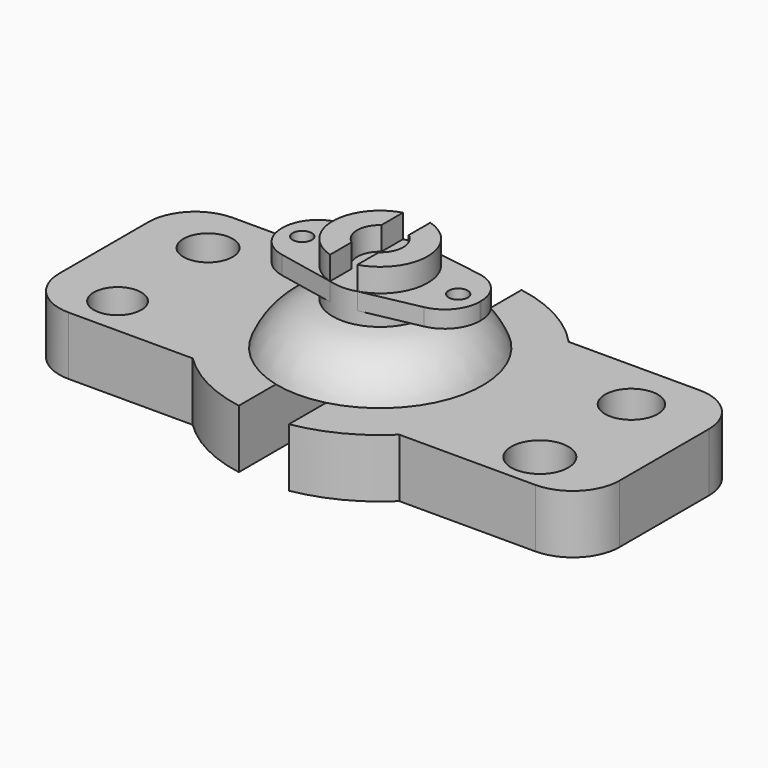
from build123d import *
from build123d import SkipClean  # not in build123d's __all__

# Parameters (mm, degrees)
F0_R      = 10.1568223354
F0_R_2    = 10.5169255504
F0_R_3    = 12.1759626717
F0_R_4    = 11.2592738499
F1_DEPTH  = 25
F2_R      = 20
F3_R      = 20
F4_R      = 20
F5_R      = 20
F6_DEPTH  = 84.25
F7_DEPTH  = 100
F8_DEPTH  = 95.25
F9_DEPTH  = 74.75
F14_DEPTH = 10
F15_DEPTH = 10
F16_DEPTH = 10
F17_DEPTH = 10
F18_DEPTH = 10
F19_R     = 4.0591498716
F20_DEPTH = 7.75
F21_R     = 15
F22_R     = 15
F23_DEPTH = 7.25
F24_R     = 15


with BuildPart() as f1:
    # F0 (on Top) → F1 (new body)
    with BuildSketch(Plane.XY):
        with BuildLine():
            Line((-46.3593495633, 42.660780251), (-117.1441823244, 42.660780251))
            Line((-117.1441823244, 42.660780251), (-117.1441823244, -44.9667572975))
            Line((-117.1441823244, -44.9667572975), (-44.1262076515, -44.9667572975))
            ThreePointArc((-44.1262076515, -44.9667572975), (-62.9805950299, -1.6050274871), (-46.3593495633, 42.660780251))
        make_face()
        with Locations((-89.4723236561, -28.3636450768)):
            Circle(F0_R, mode=Mode.SUBTRACT)
        with Locations((-89.9335220456, 20.5232948065)):
            Circle(F0_R_2, mode=Mode.SUBTRACT)
        with BuildLine():
            ThreePointArc((-10.7280304655, 62.0809215934), (-30.1500864357, 55.3182045215), (-46.3593495633, 42.660780251))
            Line((-46.3593495633, 42.660780251), (-10.7280304655, 42.660780251))
            Line((-10.7280304655, 42.660780251), (-10.7280304655, 62.0809215934))
        make_face()
        with BuildLine():
            Line((-10.7280304655, 42.660780251), (-46.3593495633, 42.660780251))
            ThreePointArc((-46.3593495633, 42.660780251), (-62.9805950299, -1.6050274871), (-44.1262076515, -44.9667572975))
            Line((-44.1262076515, -44.9667572975), (-10.7280304655, -44.9667572975))
            Line((-10.7280304655, -44.9667572975), (-10.7280304655, 42.660780251))
        make_face()
        with BuildLine():
            Line((-10.7280304655, 62.0809215934), (-10.7280304655, 42.660780251))
            Line((-10.7280304655, 42.660780251), (10.6815285981, 42.660780251))
            Line((10.6815285981, 42.660780251), (10.6815285981, 62.0889395172))
            ThreePointArc((10.6815285981, 62.0889395172), (-0.0235940182, 63.0010389349), (-10.7280304655, 62.0809215934))
        make_face()
        with BuildLine():
            Line((-10.7280304655, 68.533860147), (-10.7280304655, 62.0809215934))
            ThreePointArc((-10.7280304655, 62.0809215934), (-0.0235940182, 63.0010389349), (10.6815285981, 62.0889395172))
            Line((10.6815285981, 62.0889395172), (10.6815285981, 68.533860147))
            Line((10.6815285981, 68.533860147), (-10.7280304655, 68.533860147))
        make_face()
        with BuildLine():
            Line((-10.7280304655, -44.9667572975), (-44.1262076515, -44.9667572975))
            ThreePointArc((-44.1262076515, -44.9667572975), (-28.7310026755, -56.0683596052), (-10.7280304655, -62.0809215934))
            Line((-10.7280304655, -62.0809215934), (-10.7280304655, -44.9667572975))
        make_face()
        with BuildLine():
            Line((10.6815285981, 62.0889395172), (10.6815285981, 42.660780251))
            Line((10.6815285981, 42.660780251), (46.3593495633, 42.660780251))
            ThreePointArc((46.3593495633, 42.660780251), (30.1293675419, 55.3294919106), (10.6815285981, 62.0889395172))
        make_face()
        with BuildLine():
            Line((46.3593495633, 42.660780251), (10.6815285981, 42.660780251))
            Line((10.6815285981, 42.660780251), (10.6815285981, -44.9667572975))
            Line((10.6815285981, -44.9667572975), (44.1262076515, -44.9667572975))
            ThreePointArc((44.1262076515, -44.9667572975), (58.0910000982, -24.3837480948), (63.0010433529, 0))
            ThreePointArc((63.0010433529, 0), (58.6933507955, 22.8958956137), (46.3593495633, 42.660780251))
        make_face()
        with BuildLine():
            Line((10.6815285981, -44.9667572975), (-10.7280304655, -44.9667572975))
            Line((-10.7280304655, -44.9667572975), (-10.7280304655, -62.0809215934))
            ThreePointArc((-10.7280304655, -62.0809215934), (-0.0235940182, -63.0010389349), (10.6815285981, -62.0889395172))
            Line((10.6815285981, -62.0889395172), (10.6815285981, -44.9667572975))
        make_face()
        with BuildLine():
            ThreePointArc((10.6815285981, -62.0889395172), (-0.0235940182, -63.0010389349), (-10.7280304655, -62.0809215934))
            Line((-10.7280304655, -62.0809215934), (-10.7280304655, -71.3264122605))
            Line((-10.7280304655, -71.3264122605), (10.6815285981, -71.3264122605))
            Line((10.6815285981, -71.3264122605), (10.6815285981, -62.0889395172))
        make_face()
        with BuildLine():
            Line((122.2173571587, 42.660780251), (46.3593495633, 42.660780251))
            ThreePointArc((46.3593495633, 42.660780251), (58.6933507955, 22.8958956137), (63.0010433529, 0))
            ThreePointArc((63.0010433529, 0), (58.0910000982, -24.3837480948), (44.1262076515, -44.9667572975))
            Line((44.1262076515, -44.9667572975), (122.2173571587, -44.9667572975))
            Line((122.2173571587, -44.9667572975), (122.2173571587, 42.660780251))
        make_face()
        with Locations((90.8559188247, -28.3636450768)):
            Circle(F0_R_3, mode=Mode.SUBTRACT)
        with Locations((90.8559188247, 20.5232948065)):
            Circle(F0_R_4, mode=Mode.SUBTRACT)
        with BuildLine():
            Line((44.1262076515, -44.9667572975), (10.6815285981, -44.9667572975))
            Line((10.6815285981, -44.9667572975), (10.6815285981, -62.0889395172))
            ThreePointArc((10.6815285981, -62.0889395172), (28.7100029466, -56.079115492), (44.1262076515, -44.9667572975))
        make_face()
    extrude(amount=F1_DEPTH)

    # F2
    f2_edges = [f1.edges().sort_by_distance(p)[0] for p in [
        (-117.144182, -44.966757, 12.5),
    ]]
    fillet(f2_edges, radius=F2_R)

    # F3
    f3_edges = [f1.edges().sort_by_distance(p)[0] for p in [
        (-117.144182, 42.66078, 12.5),
    ]]
    fillet(f3_edges, radius=F3_R)

    # F4
    f4_edges = [f1.edges().sort_by_distance(p)[0] for p in [
        (122.217357, 42.66078, 12.5),
    ]]
    fillet(f4_edges, radius=F4_R)

    # F5
    f5_edges = [f1.edges().sort_by_distance(p)[0] for p in [
        (122.217357, -44.966757, 12.5),
    ]]
    fillet(f5_edges, radius=F5_R)

    # F0 (on Top) → F6 (cut)
    with BuildSketch(Plane.XY):
        with BuildLine():
            Line((-10.7280304655, 68.533860147), (-10.7280304655, 62.0809215934))
            ThreePointArc((-10.7280304655, 62.0809215934), (-0.0235940182, 63.0010389349), (10.6815285981, 62.0889395172))
            Line((10.6815285981, 62.0889395172), (10.6815285981, 68.533860147))
            Line((10.6815285981, 68.533860147), (-10.7280304655, 68.533860147))
        make_face()
    with SkipClean():  # cleaning this boolean's faces spoils the solid; the shape is the same uncleaned
        extrude(amount=F6_DEPTH, mode=Mode.SUBTRACT)

    # F0 (on Top) → F7 (cut)
    with BuildSketch(Plane.XY):
        with BuildLine():
            Line((-10.7280304655, 62.0809215934), (-10.7280304655, 42.660780251))
            Line((-10.7280304655, 42.660780251), (10.6815285981, 42.660780251))
            Line((10.6815285981, 42.660780251), (10.6815285981, 62.0889395172))
            ThreePointArc((10.6815285981, 62.0889395172), (-0.0235940182, 63.0010389349), (-10.7280304655, 62.0809215934))
        make_face()
    extrude(amount=F7_DEPTH, mode=Mode.SUBTRACT)

    # F0 (on Top) → F8 (cut)
    with BuildSketch(Plane.XY):
        with BuildLine():
            Line((10.6815285981, -44.9667572975), (-10.7280304655, -44.9667572975))
            Line((-10.7280304655, -44.9667572975), (-10.7280304655, -62.0809215934))
            ThreePointArc((-10.7280304655, -62.0809215934), (-0.0235940182, -63.0010389349), (10.6815285981, -62.0889395172))
            Line((10.6815285981, -62.0889395172), (10.6815285981, -44.9667572975))
        make_face()
    extrude(amount=F8_DEPTH, mode=Mode.SUBTRACT)

    # F0 (on Top) → F9 (cut)
    with BuildSketch(Plane.XY):
        with BuildLine():
            ThreePointArc((10.6815285981, -62.0889395172), (-0.0235940182, -63.0010389349), (-10.7280304655, -62.0809215934))
            Line((-10.7280304655, -62.0809215934), (-10.7280304655, -71.3264122605))
            Line((-10.7280304655, -71.3264122605), (10.6815285981, -71.3264122605))
            Line((10.6815285981, -71.3264122605), (10.6815285981, -62.0889395172))
        make_face()
    extrude(amount=F9_DEPTH, mode=Mode.SUBTRACT)


with BuildPart() as f11:
    # F10 (on Right) → F11 (revolve)
    with BuildSketch(Plane.YZ):
        Polygon((-20.3189048916, 25.1363171558), (0, 25.1575894654), (0, 66.0419613123), (-20.3189048916, 66.0419613123), (-20.3189048916, 43.4353500201), align=None)
    revolve(axis=Axis((0, 0, 45.5997753888), (0, 0, 1)))

    # F10 (on Right) → F12 (revolve)
    with BuildSketch(Plane.YZ):
        Polygon((-20.3189048916, 25.1363171558), (0, 25.1575894654), (0, 66.0419613123), (-20.3189048916, 66.0419613123), (-20.3189048916, 43.4353500201), align=None)
        with BuildLine():
            Line((-43.7604690051, 25.1117756655), (-20.3189048916, 25.1363171558))
            Line((-20.3189048916, 25.1363171558), (-20.3189048916, 43.4353500201))
            ThreePointArc((-20.3189048916, 43.4353500201), (-34.5417935809, 37.4745372766), (-43.7604690051, 25.1117756655))
        make_face()
    revolve(axis=Axis((0, 0, 66.0419613123), (0, 0, -1)))

    # F13 (on face) → F14 (cut)
    with BuildSketch(Plane.XY.offset(66.0419613123)):
        with BuildLine():
            Line((5.794562865, -7.9730548393), (5.794562865, 7.9730548393))
            ThreePointArc((5.794562865, 7.9730548393), (-0.028804987, 9.8562534739), (-5.8410661295, 7.9390496118))
            Line((-5.8410661295, 7.9390496118), (-5.8410661295, -7.9390496118))
            ThreePointArc((-5.8410661295, -7.9390496118), (-0.028804987, -9.8562534739), (5.794562865, -7.9730548393))
        make_face()
    extrude(amount=-F14_DEPTH, mode=Mode.SUBTRACT)

    # F13 (on face) → F15 (cut)
    with BuildSketch(Plane.XY.offset(66.0419613123)):
        with BuildLine():
            ThreePointArc((-5.8410661295, 7.9390496118), (-0.028804987, 9.8562534739), (5.794562865, 7.9730548393))
            Line((5.794562865, 7.9730548393), (5.794562865, 19.4751363846))
            ThreePointArc((5.794562865, 19.4751363846), (-0.0242676601, 20.3188903997), (-5.8410661295, 19.4612394894))
            Line((-5.8410661295, 19.4612394894), (-5.8410661295, 7.9390496118))
        make_face()
    extrude(amount=-F15_DEPTH, mode=Mode.SUBTRACT)

    # F13 (on face) → F16 (cut)
    with BuildSketch(Plane.XY.offset(66.0419613123)):
        with BuildLine():
            Line((5.794562865, -19.4751363846), (5.794562865, -7.9730548393))
            ThreePointArc((5.794562865, -7.9730548393), (-0.028804987, -9.8562534739), (-5.8410661295, -7.9390496118))
            Line((-5.8410661295, -7.9390496118), (-5.8410661295, -19.4612394894))
            ThreePointArc((-5.8410661295, -19.4612394894), (-0.0242676601, -20.3188903997), (5.794562865, -19.4751363846))
        make_face()
    extrude(amount=-F16_DEPTH, mode=Mode.SUBTRACT)

    # F13 (on face) → F17 (cut)
    with BuildSketch(Plane.XY.offset(66.0419613123)):
        with BuildLine():
            Line((-5.8410661295, -7.9390496118), (-5.8410661295, 7.9390496118))
            ThreePointArc((-5.8410661295, 7.9390496118), (-9.8562955652, 0), (-5.8410661295, -7.9390496118))
        make_face()
    extrude(amount=-F17_DEPTH, mode=Mode.SUBTRACT)

    # F13 (on face) → F18 (cut)
    with BuildSketch(Plane.XY.offset(66.0419613123)):
        with BuildLine():
            ThreePointArc((5.794562865, -7.9730548393), (8.7823540847, -4.4740159812), (9.8562955652, 0))
            ThreePointArc((9.8562955652, 0), (8.7823540847, 4.4740159812), (5.794562865, 7.9730548393))
            Line((5.794562865, 7.9730548393), (5.794562865, -7.9730548393))
        make_face()
    extrude(amount=-F18_DEPTH, mode=Mode.SUBTRACT)

    # F19 (on face) → F20 (join)
    with BuildSketch(Plane.XY.offset(56.0419613123)):
        with BuildLine():
            Line((-5.8410661295, 7.9390496118), (-5.8410661295, 19.4612394894))
            Line((-5.8410661295, 19.4612394894), (-42.3769466579, 13.7001445506))
            Line((-42.3769466579, 13.7001445506), (-42.3769466579, -12.0281800628))
            Line((-42.3769466579, -12.0281800628), (-5.8410661295, -19.4612394894))
            Line((-5.8410661295, -19.4612394894), (-5.8410661295, -7.9390496118))
            ThreePointArc((-5.8410661295, -7.9390496118), (-9.8562955652, 0), (-5.8410661295, 7.9390496118))
        make_face()
        with Locations((-33.3011560142, 0)):
            Circle(F19_R, mode=Mode.SUBTRACT)
    extrude(amount=-F20_DEPTH)

    # F21
    f21_edges = [f11.edges().sort_by_distance(p)[0] for p in [
        (-42.376947, -12.02818, 52.166961),
    ]]
    fillet(f21_edges, radius=F21_R)

    # F22
    f22_edges = [f11.edges().sort_by_distance(p)[0] for p in [
        (-42.376947, 13.700145, 52.166961),
    ]]
    fillet(f22_edges, radius=F22_R)

    # F19 (on face) → F23 (join)
    with BuildSketch(Plane.XY.offset(56.0419613123)):
        with BuildLine():
            Line((5.8410661295, 19.4612394894), (5.794562865, 7.9730548393))
            ThreePointArc((5.794562865, 7.9730548393), (10.5983419931, 0), (5.794562865, -7.9730548393))
            Line((5.794562865, -7.9730548393), (5.8410661295, -19.4612394894))
            Line((5.8410661295, -19.4612394894), (42.3769466579, -12.0281800628))
            Line((42.3769466579, -12.0281800628), (42.3769466579, 13.7001445506))
            Line((42.3769466579, 13.7001445506), (5.8410661295, 19.4612394894))
        make_face()
        with Locations((33.3011560142, 0)):
            Circle(F19_R, mode=Mode.SUBTRACT)
    extrude(amount=-F23_DEPTH)

    # F24
    f24_edges = [f11.edges().sort_by_distance(p)[0] for p in [
        (42.376947, 13.700145, 52.416961),
        (42.376947, -12.02818, 52.416961),
    ]]
    fillet(f24_edges, radius=F24_R)


solid = Compound([f1.part, f11.part])
